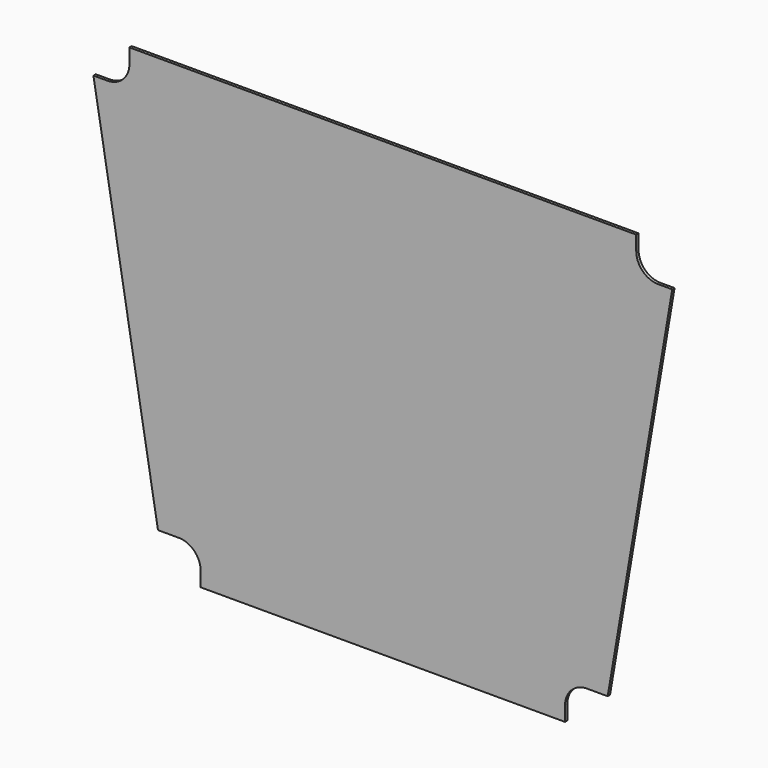
from build123d import *

# Parameters (mm, degrees)
F1_DEPTH = 1.6
F2_W     = 400.5107134581
F2_H     = 323.6893676221
F3_DEPTH = 25
F4_W     = 46.074695995
F4_H     = 35.5617606323
F5_DEPTH = 25
F6_W     = 59.3347663573
F6_H     = 53.373508143
F7_DEPTH = 25
F8_R     = 12


# Not quite as in the source:
# - a pattern or mirror of a feature is missing from the dataset's text; its kind, count and spacing are read off the source's solid


with BuildPart() as f1:
    # F0 (on Front) → F1 (new body)
    with BuildSketch(Plane.XZ):
        Polygon((165, 30.1805247461), (-165, 30.1805247461), (-165, 5.1805247461), (-125, -229.8194752539), (125, -229.8194752539), (165, 5.1805247461), align=None)
    extrude(amount=F1_DEPTH)

    # F2 (on face) → F3 (cut)
    with BuildSketch(Plane.XZ.offset(1.6)):
        with Locations((5.1858350635, -103.1377185136)):
            Rectangle(F2_W, F2_H)
        Polygon((-159, 5.6875170693), (-159, 24.1805247461), (159, 24.1805247461), (159, 5.6875170693), (119.9349800301, -223.8194752539), (-119.9349800301, -223.8194752539), align=None, mode=Mode.SUBTRACT)
    extrude(amount=-F3_DEPTH, mode=Mode.SUBTRACT)

    # F4 (on face) → F5 (cut)
    with BuildSketch(Plane.XZ.offset(1.6)):
        with Locations((162.0373479975, 21.9614050622)):
            Rectangle(F4_W, F4_H)
    f5 = extrude(amount=-F5_DEPTH, mode=Mode.SUBTRACT)

    # F5_copies: F5 across plane
    add(f5.mirror(Plane(origin=(0, 0, 0), x_dir=(0, 0, -1), z_dir=(-1, 0, 0))), mode=Mode.SUBTRACT)

    # F6 (on face) → F7 (cut)
    with BuildSketch(Plane.XZ.offset(1.6)):
        with Locations((129.6023632087, -230.5062293254)):
            Rectangle(F6_W, F6_H)
    f7 = extrude(amount=-F7_DEPTH, mode=Mode.SUBTRACT)

    # F7_copies: F7 across plane
    add(f7.mirror(Plane(origin=(0, 0, 0), x_dir=(0, 0, -1), z_dir=(-1, 0, 0))), mode=Mode.SUBTRACT)

    # F8
    f8_edges = [f1.edges().sort_by_distance(p)[0] for p in [
        (139, -0.8, 4.180525),
        (99.93498, -0.8, -203.819475),
        (-99.93498, -0.8, -203.819475),
        (-139, -0.8, 4.180525),
    ]]
    fillet(f8_edges, radius=F8_R)


solid = f1.part
